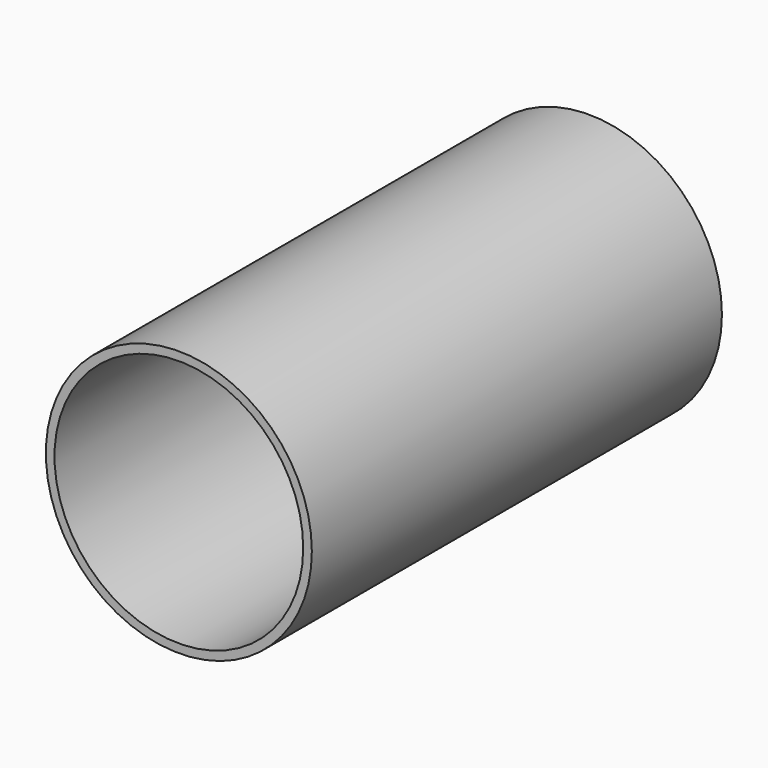
from build123d import *

# Parameters (mm, degrees)
F0_R     = 39.5391392568
F1_DEPTH = 152.4
F2_R     = 36.9688398978
F3_DEPTH = 132.588


# Not quite as in the source:
# - a feature names something its author has since deleted; it is built from what else it names


with BuildPart() as f1:
    # F0 (on Front) → F1 (new body)
    with BuildSketch(Plane.XZ):
        Circle(F0_R)
    extrude(amount=F1_DEPTH)

    # F2 (on face) → F3 (cut)
    with BuildSketch(Plane.XZ.offset(152.4)):
        Circle(F2_R)
    extrude(amount=-F3_DEPTH, mode=Mode.SUBTRACT)


solid = f1.part
